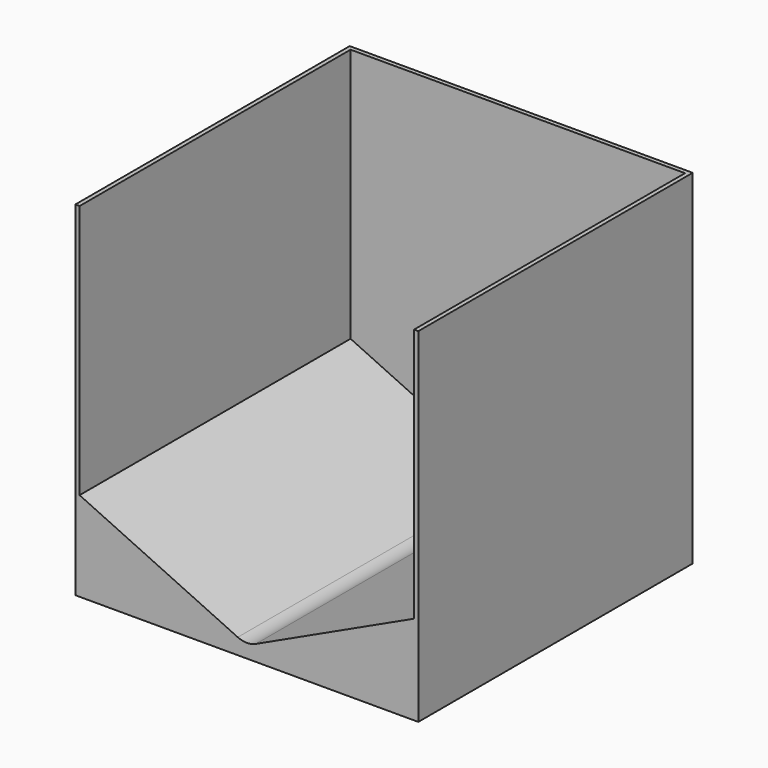
from build123d import *

# Parameters (mm, degrees)
F1_DEPTH     = 100
F2_T         = -2.5
F3_R         = 5
F4_DEPTH     = 200.001
F6_DEPTH     = 200
F7_T         = 10
F7_T3_DEPTH  = 168.4060893131
F7_T5_DEPTH  = 121.7259809119
F7_T7_DEPTH  = 121.7259809119
F7_T9_DEPTH  = 217.5
F7_T12_ANGLE = 49.9194838504


# Not quite as in the source:
# - a shell that OpenCascade refuses in one call is made with other operations: the cavity is built on its own and cut out


with BuildPart() as f1:
    # F0 (on Front) → F1 (new body, symmetric)
    with BuildSketch(Plane.XZ):
        with BuildLine():
            Line((200, 150), (0, 150))
            Line((0, 150), (0, 0))
            Line((0, 0), (93.6702797046, -43.5990676512))
            ThreePointArc((93.6702797046, -43.5990676512), (91.9360618935, -17.3519605387), (115, -30))
            ThreePointArc((115, -30), (112.6480394613, -38.0639381065), (106.3297202954, -43.5990676512))
            Line((106.3297202954, -43.5990676512), (200, 0))
            Line((200, 0), (200, 150))
        make_face()
        with BuildLine():
            ThreePointArc((115, -30), (91.9360618935, -17.3519605387), (93.6702797046, -43.5990676512))
            ThreePointArc((93.6702797046, -43.5990676512), (100, -45), (106.3297202954, -43.5990676512))
            ThreePointArc((106.3297202954, -43.5990676512), (112.6480394613, -38.0639381065), (115, -30))
        make_face()
    extrude(amount=F1_DEPTH, both=True)

    # F2
    f2_openings = [f1.faces().sort_by_distance(p)[0] for p in [
        (100, -100, 62.86367),
        (100, 0, 150),
    ]]
    offset(amount=F2_T, openings=f2_openings)

    # F3 (on face) → F4 (cut, through all)
    with BuildSketch(Plane(origin=(0, 100, 0), x_dir=(-1, 0, 0), z_dir=(0, 1, 0))):
        with Locations((-100, -35)):
            Circle(F3_R)
    extrude(amount=-F4_DEPTH, mode=Mode.SUBTRACT)

    # F5 (on face) → F6 (join)
    with BuildSketch(Plane.XZ.offset(100)):
        with BuildLine():
            Line((93.6702797046, -43.5990676512), (0, 0))
            Line((0, 0), (0, -50.5793318152))
            Line((0, -50.5793318152), (200, -50.5793318152))
            Line((200, -50.5793318152), (200, 0))
            Line((200, 0), (106.3297202954, -43.5990676512))
            ThreePointArc((106.3297202954, -43.5990676512), (103.2414491537, -44.64557979), (100, -45))
            ThreePointArc((100, -45), (96.7585508463, -44.64557979), (93.6702797046, -43.5990676512))
        make_face()
    extrude(amount=-F6_DEPTH)

    # F7: shell of thickness 10, made by hand


with BuildPart() as f7_core1:
    # F7_t2: copy of F1
    add(f1.part)

    # the walls: a layer under each face that stays
    f7_faces = [f7_core1.faces().sort_by_distance(p)[0] for p in [
        (200, 0, 49.7103340924),
        (100, 100, 49.7103340924),
        (105, 98.75, -35),
        (100, 97.5, 53.75),
        (100, -1.25, -42.5),
        (48.6126165436, -1.25, -19.8693228445),
        (151.3873834564, -1.25, -19.8693228445),
        (2.5, -1.25, 75.7969553435),
        (197.5, -1.25, 75.7969553435),
        (0, 0, 49.7103340924),
        (33.3333333333, -100, -17.1494431794),
        (31.25, 97.5308641975, 150),
    ]]
    thicken(f7_faces, amount=-F7_T, mode=Mode.SUBTRACT)

    # F7_s4 → F7_t3 (cut)
    with BuildSketch(Plane.XY.offset(-8.4060893131)):
        Polygon((197.4, 97.4), (197.5, 107.5), (207.5, 107.5), (207.5, 97.5), align=None)
        Polygon((2.6, 97.4), (2.5, 107.5), (-7.5, 107.5), (-7.5, 97.5), align=None)
    extrude(amount=F7_T3_DEPTH, mode=Mode.SUBTRACT)

    # F7_s6 → F7_t5 (cut)
    with BuildSketch(Plane(origin=(61.6500227345, 0, 28.695158383), x_dir=(0, 1, 0), z_dir=(0.9066045101, 0, 0.421981353))):
        Polygon((97.4, -81.7962706049), (107.5, -81.8962706049), (107.5, -91.8962706049), (97.5, -91.8962706049), align=None)
    extrude(amount=F7_T5_DEPTH, mode=Mode.SUBTRACT)

    # F7_s8 → F7_t7 (cut)
    with BuildSketch(Plane(origin=(-7.6209984834, 0, 3.547212942), x_dir=(0, 1, 0), z_dir=(0.9066045101, 0, -0.421981353))):
        Polygon((97.4, 2.6), (107.5, 2.5), (107.5, -7.5), (97.5, -7.5), align=None)
    extrude(amount=F7_T7_DEPTH, mode=Mode.SUBTRACT)

    # F7_s10 → F7_t9 (cut)
    with BuildSketch(Plane.XZ.offset(-107.5)):
        Polygon((2.6421981353, 1.6845711379), (-1.7198135302, -7.4721344139), (-7.5, -4.7817320608), (-7.5, 1.5939106869), align=None)
        Polygon((197.3578018647, 1.6845711379), (201.7198135302, -7.4721344139), (207.5, -4.7817320608), (207.5, 1.5939106869), align=None)
    extrude(amount=F7_T9_DEPTH, mode=Mode.SUBTRACT)

    # F7_s11 → F7_t12 (revolve, cut)
    with BuildSketch(Plane(origin=(93.6702797046, 0, -43.5990676512), x_dir=(0, 1, 0), z_dir=(-0.9066045101, 0, 0.421981353))):
        Polygon((97.4, -2.6), (107.5, -2.5), (107.5, 7.5), (97.5, 7.5), align=None)
    revolve(axis=Axis((100, 97.5, -30), (0, -1, 0)), revolution_arc=F7_T12_ANGLE, mode=Mode.SUBTRACT)


with BuildPart() as f1_1:
    add(f1.part)

    # what is left inside the walls is the cavity
    f7_cavity = [f7_core1.part.solids().sort_by_distance(p)[0] for p in [
        (149.789488, 30, -31.753537),
        (50.210512, 30, -31.753537),
    ]]
    add(f7_cavity, mode=Mode.SUBTRACT)


solid = f1_1.part
